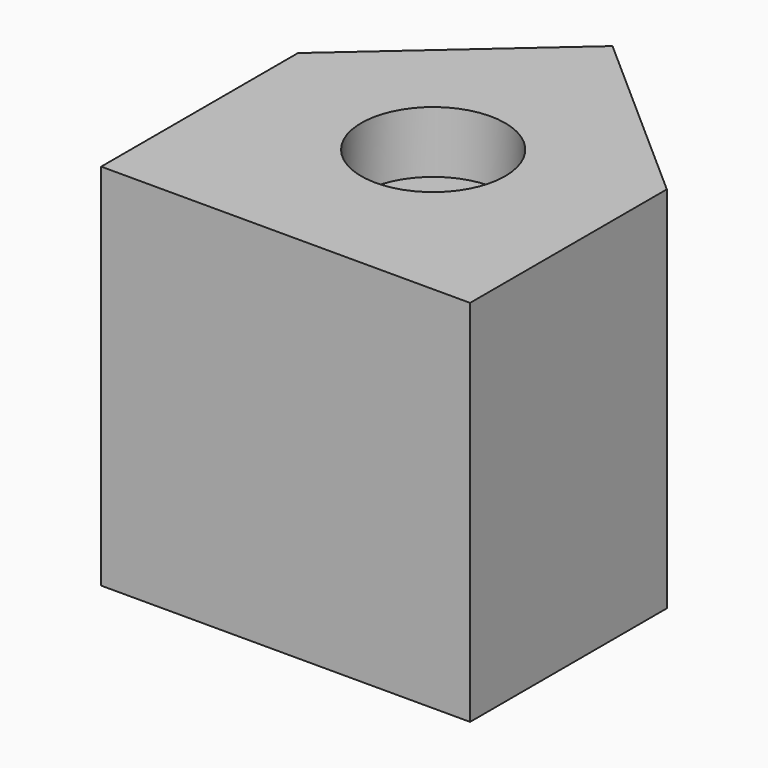
from build123d import *

# Parameters (mm, degrees)
F0_R     = 11.7054565065
F1_DEPTH = 60
F2_START = 10
F2_DEPTH = 40


# Not quite as in the source:
# - a feature names something its author has since deleted; it is built from what else it names


with BuildPart() as f1:
    # F0 (on Top) → F1 (new body)
    with BuildSketch(Plane.XY):
        Polygon((-60, 40.0004889347), (-60, 0), (0, 0), (0, 40), (-29.9997844001, 66.457757576), align=None)
        with Locations((-29.9997844001, 30)):
            Circle(F0_R, mode=Mode.SUBTRACT)
    extrude(amount=F1_DEPTH)

    # F0 (on Top) → F2 (join)
    with BuildSketch(Plane.XY.offset(F2_START)):
        with Locations((-29.9997844001, 30)):
            Circle(F0_R)
    extrude(amount=F2_DEPTH)


solid = f1.part
